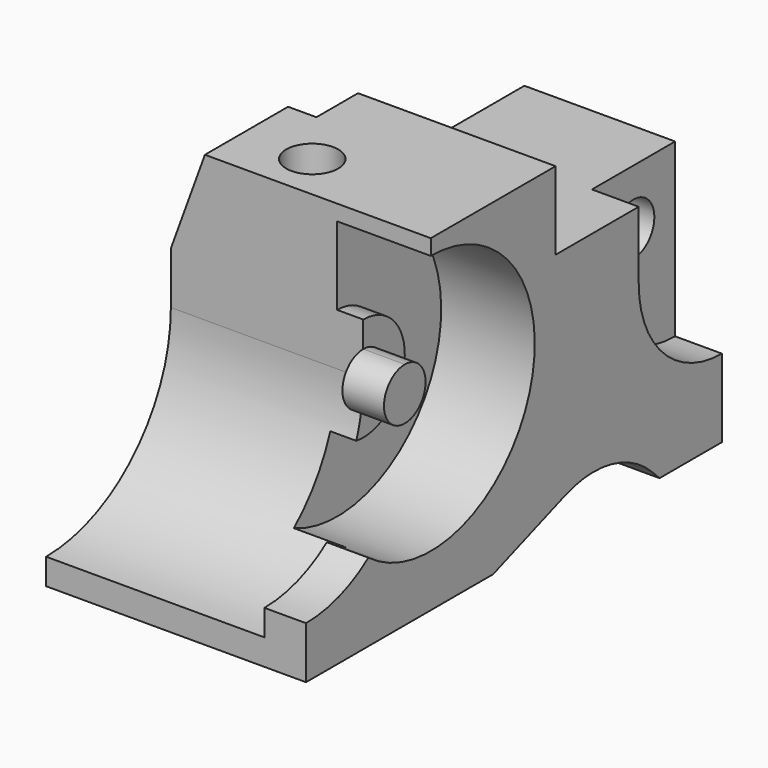
from build123d import *

# Parameters (mm, degrees)
F0_W      = 100
F0_H      = 63
F1_DEPTH  = 50
F3_DEPTH  = 50.001
F4_W      = 40
F4_H      = 15
F5_DEPTH  = 50.001
F7_DEPTH  = 9
F8_R      = 5
F9_DEPTH  = 41.001
F10_W     = 12
F10_H     = 10
F10_H_2   = 40
F11_DEPTH = 63.001
F13_DEPTH = 187
F15_DEPTH = 100.001
F16_R     = 25
F17_DEPTH = 18
F18_R     = 10
F19_DEPTH = 5
F22_DEPTH = 42
F20_R     = 25
F23_DEPTH = 8
F25_DEPTH = 8
F26_W     = 40
F26_H     = 9
F27_DEPTH = 8.001
F28_R     = 5
F29_DEPTH = 63.001


# Not quite as in the source:
# - an extrude ends at something that could not be found from the text; its depth is read off the source's solid


with BuildPart() as f1:
    # F0 (on Right) → F1 (new body)
    with BuildSketch(Plane.YZ):
        with Locations((50, 31.5)):
            Rectangle(F0_W, F0_H)
    extrude(amount=F1_DEPTH)

    # F2 (on face) → F3 (cut, through all)
    with BuildSketch(Plane.YZ.offset(50)):
        with BuildLine():
            Line((62.353148703, 6.3160295987), (45, 0))
            Line((45, 0), (85, 0))
            Line((85, 0), (83.3356871933, 1.6643128067))
            ThreePointArc((83.3356871933, 1.6643128067), (73.5223438483, 7.0480973254), (62.353148703, 6.3160295987))
        make_face()
    extrude(amount=-F3_DEPTH, mode=Mode.SUBTRACT)

    # F4 (on face) → F5 (cut, through all)
    with BuildSketch(Plane.YZ.offset(50)):
        with Locations((80, 55.5)):
            Rectangle(F4_W, F4_H)
    extrude(amount=-F5_DEPTH, mode=Mode.SUBTRACT)

    # F6 (on face) → F7 (cut)
    with BuildSketch(Plane.YZ.offset(50)):
        with BuildLine():
            ThreePointArc((84.8013158464, 48), (81.2386876382, 41.9291527956), (80, 35))
            ThreePointArc((80, 35), (85.8578643763, 20.8578643763), (100, 15))
            Line((100, 15), (100, 48))
            Line((100, 48), (84.8013158464, 48))
        make_face()
        with BuildLine():
            Line((80, 48), (80, 35))
            ThreePointArc((80, 35), (81.2386876382, 41.9291527956), (84.8013158464, 48))
            Line((84.8013158464, 48), (80, 48))
        make_face()
    extrude(amount=-F7_DEPTH, mode=Mode.SUBTRACT)

    # F8 (on face) → F9 (cut, through all)
    with BuildSketch(Plane.YZ.offset(41)):
        with Locations((90, 37.2308082879)):
            Circle(F8_R)
    extrude(amount=-F9_DEPTH, mode=Mode.SUBTRACT)

    # F10 (on face) → F11 (cut, through all)
    with BuildSketch(Plane.XY.offset(63)):
        with Locations((6, 55)):
            Rectangle(F10_W, F10_H)
        with Locations((6, 80)):
            Rectangle(F10_W, F10_H_2)
    extrude(amount=-F11_DEPTH, mode=Mode.SUBTRACT)

    # F12 (on face) → F13 (cut, through all)
    with BuildSketch(Plane.XZ):
        Polygon((0, 63), (0, 45), (6.5514642168, 63), align=None)
    extrude(amount=F13_DEPTH, mode=Mode.SUBTRACT)

    # F14 (on face) → F15 (cut, through all)
    with BuildSketch(Plane.XZ):
        Polygon((0, 63), (0, 45), (6.5514642168, 63), align=None)
    extrude(amount=-F15_DEPTH, mode=Mode.SUBTRACT)

    # F16 (on face) → F17 (cut)
    with BuildSketch(Plane.YZ.offset(50)):
        with Locations((30, 35)):
            Circle(F16_R)
    extrude(amount=-F17_DEPTH, mode=Mode.SUBTRACT)

    # F18 (on face) → F19 (join)
    with BuildSketch(Plane.YZ.offset(32)):
        with Locations((30, 35)):
            Circle(F18_R)
    extrude(amount=F19_DEPTH)

    # F21 (on face) → F22 (cut)
    with BuildSketch(Plane(origin=(0, 0, 0), x_dir=(0, -1, 0), z_dir=(-1, 0, 0))):
        with BuildLine():
            Line((-30, 63), (-30, 35))
            ThreePointArc((-30, 35), (21.9316580473, 14.5304524892), (-2.0665083135, 64.9287410926))
            Line((-2.0665083135, 64.9287410926), (-30, 63))
        make_face()
    extrude(amount=-F22_DEPTH, mode=Mode.SUBTRACT)

    # F20 (on face) → F23 (cut)
    with BuildSketch(Plane.YZ.offset(50)):
        with Locations((0, 35)):
            Circle(F20_R)
    extrude(amount=-F23_DEPTH, mode=Mode.SUBTRACT)

    # F24 (on face) → F25 (join)
    with BuildSketch(Plane.YZ.offset(37)):
        with BuildLine():
            ThreePointArc((29.5833333333, 30.017391357), (33.3850160019, 31.320099639), (35, 35))
            ThreePointArc((35, 35), (33.5355339059, 38.5355339059), (30, 40))
            Line((30, 40), (30, 35))
            ThreePointArc((30, 35), (29.8956518578, 32.5), (29.5833333333, 30.017391357))
        make_face()
        with BuildLine():
            Line((30, 35), (30, 40))
            ThreePointArc((30, 40), (25.0043497313, 35.2085147299), (29.5833333333, 30.017391357))
            ThreePointArc((29.5833333333, 30.017391357), (29.8956518578, 32.5), (30, 35))
        make_face()
    extrude(amount=F25_DEPTH)

    # F26 (on face) → F27 (cut, through all)
    with BuildSketch(Plane(origin=(42, 0, 0), x_dir=(0, -1, 0), z_dir=(-1, 0, 0))):
        with Locations((-10, 58.5)):
            Rectangle(F26_W, F26_H)
    extrude(amount=-F27_DEPTH, mode=Mode.SUBTRACT)

    # F28 (on face) → F29 (cut, through all)
    with BuildSketch(Plane.XY.offset(63)):
        with Locations((20, 39)):
            Circle(F28_R)
    extrude(amount=-F29_DEPTH, mode=Mode.SUBTRACT)


solid = f1.part
